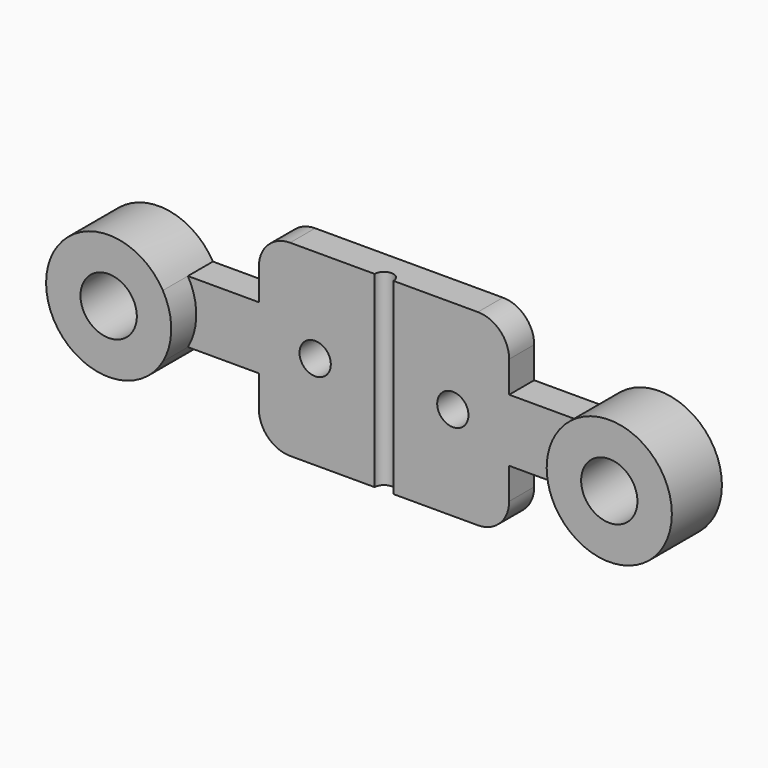
from build123d import *

# Parameters (mm, degrees)
F0_W     = 15
F0_H     = 10
F0_R     = 2.5
F1_DEPTH = 5
F3_DEPTH = 31
F4_R     = 4.5
F5_DEPTH = 10
F6_R     = 5


# Not quite as in the source:
# - a feature names something its author has since deleted; it is built from what else it names


with BuildPart() as f1:
    # F0 (on Front) → F1 (new body)
    with BuildSketch(Plane.XZ):
        with Locations((-27.5, 0)):
            Rectangle(F0_W, F0_H)
        Polygon((20, 15), (-20, 15), (-20, 5), (-20, -5), (-20, -15), (20, -15), (20, -5), (20, 5), align=None)
        with Locations((-11, 0)):
            Circle(F0_R, mode=Mode.SUBTRACT)
        with Locations((11, 0)):
            Circle(F0_R, mode=Mode.SUBTRACT)
        with Locations((27.5, 0)):
            Rectangle(F0_W, F0_H)
    extrude(amount=F1_DEPTH)

    # F2 (on face) → F3 (cut)
    with BuildSketch(Plane(origin=(0, 0, -15), x_dir=(1, 0, 0), z_dir=(0, 0, -1))):
        with BuildLine():
            ThreePointArc((-1.5, 5), (0, 3.5), (1.5, 5))
            Line((1.5, 5), (-1.5, 5))
        make_face()
    extrude(amount=-F3_DEPTH, mode=Mode.SUBTRACT)

    # F4 (on face) → F5 (join)
    with BuildSketch(Plane(origin=(0, 0, 0), x_dir=(-1, 0, 0), z_dir=(0, 1, 0))):
        with BuildLine():
            ThreePointArc((50, 0), (42.588190451, 9.6592582629), (31.3397459622, 5))
            Line((31.3397459622, 5), (35, 5))
            Line((35, 5), (35, -5))
            Line((35, -5), (31.3397459622, -5))
            ThreePointArc((31.3397459622, -5), (42.588190451, -9.6592582629), (50, 0))
        make_face()
        with Locations((40, 0)):
            Circle(F4_R, mode=Mode.SUBTRACT)
        with BuildLine():
            Line((-35, 5), (-31.3397459622, 5))
            ThreePointArc((-31.3397459622, 5), (-50, 0), (-31.3397459622, -5))
            Line((-31.3397459622, -5), (-35, -5))
            Line((-35, -5), (-35, 5))
        make_face()
        with Locations((-40, 0)):
            Circle(F4_R, mode=Mode.SUBTRACT)
        with BuildLine():
            ThreePointArc((-31.3397459622, -5), (-30.3407417371, -2.588190451), (-30, 0))
            ThreePointArc((-30, 0), (-30.3407417371, 2.588190451), (-31.3397459622, 5))
            Line((-31.3397459622, 5), (-35, 5))
            Line((-35, 5), (-35, -5))
            Line((-35, -5), (-31.3397459622, -5))
        make_face()
        with BuildLine():
            Line((35, 5), (31.3397459622, 5))
            ThreePointArc((31.3397459622, 5), (30, 0), (31.3397459622, -5))
            Line((31.3397459622, -5), (35, -5))
            Line((35, -5), (35, 5))
        make_face()
    extrude(amount=-F5_DEPTH)

    # F6
    f6_edges = [f1.edges().sort_by_distance(p)[0] for p in [
        (20, -2.5, -15),
        (20, -2.5, 15),
        (-20, -2.5, 15),
        (-20, -2.5, -15),
    ]]
    fillet(f6_edges, radius=F6_R)


solid = f1.part
